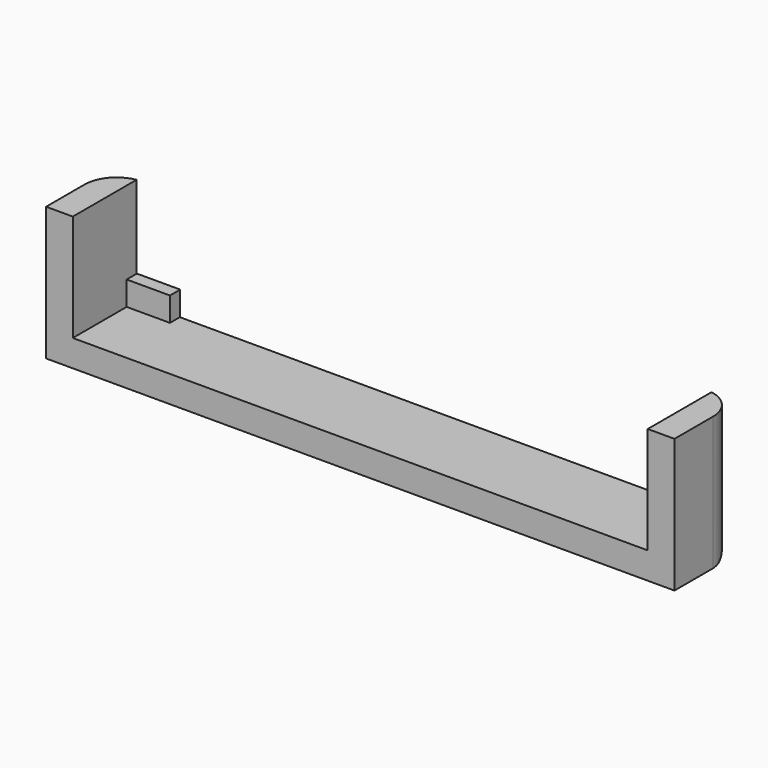
from build123d import *

# Parameters (mm, degrees)
F1_DEPTH    = 19.05
F2_W        = 10.287
F2_H        = 5.9704589657
F2_W_2      = 10.7644796371
F3_DEPTH    = 3.048
F4_T1_DEPTH = 69.8499994576
F4_T3_DEPTH = 187.4519989152


# Not quite as in the source:
# - a fillet or chamfer that OpenCascade refuses, or shapes differently, is made with other operations: its cross-section is extruded or revolved along the edge and cut away or added


with BuildPart() as f1:
    # F0 (on Front) → F1 (new body)
    with BuildSketch(Plane.XZ):
        Polygon((-38.0874201655, -5.7323638652), (-38.0874201655, 19.6676361348), (-44.4374196231, 19.6676361348), (-44.4374196231, -12.0823633227), (104.9145792921, -12.0823633227), (104.9145792921, 19.6676361348), (98.5645798345, 19.6676361348), (98.5645798345, -5.7323638652), align=None)
    extrude(amount=F1_DEPTH)

    # F2 (on Front) → F3 (join)
    with BuildSketch(Plane.XZ):
        with Locations((-32.9439201655, -2.9852294829)):
            Rectangle(F2_W, F2_H)
        with Locations((93.29213202, -2.9852294829)):
            Rectangle(F2_W_2, F2_H)
    extrude(amount=F3_DEPTH)

    # F4: fillet of radius 7.62 on 3 edges, made by hand

    # F4_s2 → F4_t1 (cut)
    with BuildSketch(Plane.XY.offset(-31.1323633227)):
        with BuildLine():
            ThreePointArc((97.2945792921, 0), (102.6827329647, -2.2318463274), (104.9145792921, -7.62))
            Line((104.9145792921, -7.62), (104.9145792921, 0))
            Line((104.9145792921, 0), (97.2945792921, 0))
        make_face()
        with BuildLine():
            ThreePointArc((-36.8174196231, 0), (-42.2055732958, -2.2318463274), (-44.4374196231, -7.62))
            Line((-44.4374196231, -7.62), (-44.4374196231, 0))
            Line((-44.4374196231, 0), (-36.8174196231, 0))
        make_face()
    extrude(amount=F4_T1_DEPTH, mode=Mode.SUBTRACT)

    # F4_s4 → F4_t3 (cut)
    with BuildSketch(Plane.YZ.offset(-63.4874196231)):
        with BuildLine():
            ThreePointArc((0, -4.4623633227), (-2.2318463274, -9.8505169954), (-7.62, -12.0823633227))
            Line((-7.62, -12.0823633227), (0, -12.0823633227))
            Line((0, -12.0823633227), (0, -4.4623633227))
        make_face()
    extrude(amount=F4_T3_DEPTH, mode=Mode.SUBTRACT)


solid = f1.part
